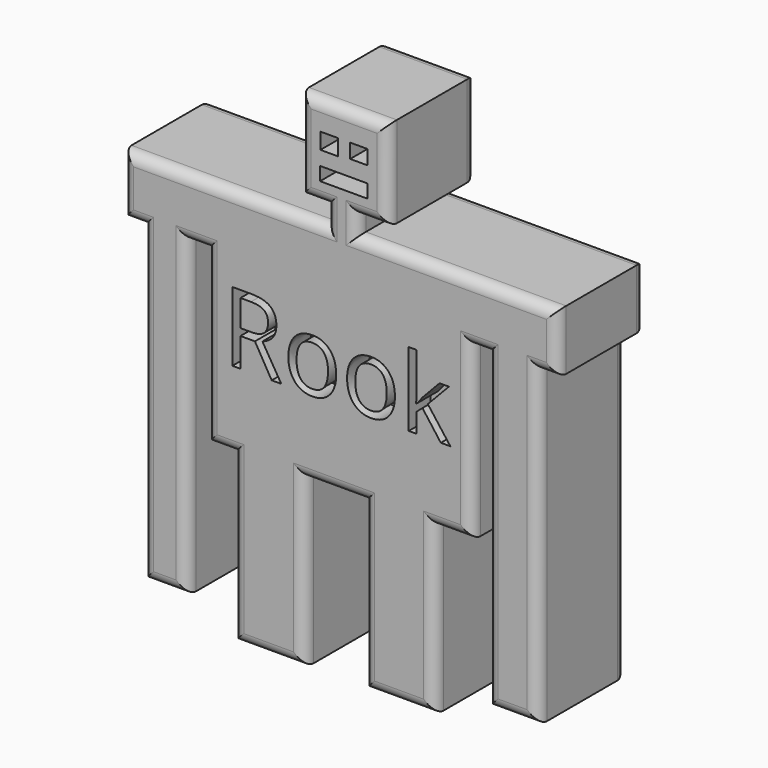
from build123d import *

# Parameters (mm, degrees)
F0_W         = 7.1803850587
F0_H         = 4.1030719876
F0_W_2       = 10.2576911449
F0_H_2       = 72.1457730979
F0_W_3       = 11.7963477969
F0_W_4       = 16.5832703933
F0_H_3       = 38.4663501754
F0_W_5       = 16.4123084396
F0_H_4       = 38.2953854278
F1_DEPTH     = 25.4
F2_R         = 2.54
F3_TEXT_SIZE = 22.484323967
F4_DEPTH     = 6.35
F5_W         = 4.116662778
F5_H         = 3.7231482565
F5_W_2       = 4.0594090242
F5_H_2       = 3.3319927752
F5_W_3       = 10.9823788516
F5_H_3       = 3.1074360013
F6_DEPTH     = 6.35


# Not quite as in the source:
# - a length typed as a fraction of an inch, garbled in the dataset ("3 / 203.2 mm" for 3/8 in), is restored
# - Text() gives the source's letters only with a copy of the font that has no kerning and outlines rounded to 1/6400 em; it was checked with that copy


with BuildPart() as f1:
    # F0 (on Front) → F1 (new body)
    with BuildSketch(Plane.XZ):
        Polygon((11.5399044007, 63.8541355729), (-8.8045196608, 63.8541355729), (-8.8045196608, 42.8258627653), (-2.820865484, 42.8258627653), (4.3595195748, 42.8258627653), (11.5399044007, 42.8258627653), align=None)
        with Locations((0.7693270454, 40.7743267715)):
            Rectangle(F0_W, F0_H)
        Polygon((4.3595195748, 38.7227907777), (-2.820865484, 38.7227907777), (-30.5166337639, 38.7227907777), (-30.5166337639, 24.8749051243), (-30.5166337639, -14.6172111854), (-24.3620201945, -14.6172111854), (-7.7787498012, -14.6172111854), (5.8981720358, -14.6172111854), (22.3104804754, -14.6172111854), (30.858559534, -14.6172111854), (30.858559534, 24.8749051243), (30.858559534, 38.7227907777), align=None)
        Polygon((-30.5166337639, 24.8749051243), (-30.5166337639, 38.7227907777), (-49.8352870345, 38.7227907777), (-49.8352870345, 24.8749051243), (-45.2193245292, 24.8749051243), (-34.9616333842, 24.8749051243), align=None)
        Polygon((50.6900958717, 38.7227907777), (30.858559534, 38.7227907777), (30.858559534, 24.8749051243), (34.4487503171, 24.8749051243), (46.245098114, 24.8749051243), (50.6900958717, 24.8749051243), align=None)
        with Locations((-40.0904789567, -11.1979814246)):
            Rectangle(F0_W_2, F0_H_2)
        with Locations((40.3469242156, -11.1979814246)):
            Rectangle(F0_W_3, F0_H_2)
        with Locations((-16.0703849979, -33.8503862731)):
            Rectangle(F0_W_4, F0_H_3)
        with Locations((14.1043262556, -33.7649038993)):
            Rectangle(F0_W_5, F0_H_4)
    extrude(amount=-F1_DEPTH)

    # F2
    f2_edges = [f1.edges().sort_by_distance(p)[0] for p in [
        (1.367692, 0, 63.854136),
        (-8.80452, 0, 53.339999),
        (-5.812693, 0, 42.825863),
        (-2.820865, 0, 40.774327),
        (-26.328076, 0, 38.722791),
        (-49.835287, 0, 31.798848),
        (-47.527306, 0, 24.874905),
        (-45.219325, 0, -11.197981),
        (-40.090479, 0, -47.270868),
        (-34.961633, 0, -11.197981),
        (-32.739134, 0, 24.874905),
        (-30.516634, 0, 5.128847),
        (-27.439327, 0, -14.617211),
        (-24.36202, 0, -33.850386),
        (-16.070385, 0, -53.083561),
        (-7.77875, 0, -33.850386),
        (-0.940289, 0, -14.617211),
        (5.898172, 0, -33.764904),
        (14.104326, 0, -52.912597),
        (22.31048, 0, -33.764904),
        (26.58452, 0, -14.617211),
        (30.85856, 0, 5.128847),
        (32.653655, 0, 24.874905),
        (34.44875, 0, -11.197981),
        (40.346924, 0, -47.270868),
        (46.245098, 0, -11.197981),
        (48.467597, 0, 24.874905),
        (50.690096, 0, 31.798848),
        (27.524808, 0, 38.722791),
        (4.35952, 0, 40.774327),
        (7.949712, 0, 42.825863),
        (11.539904, 0, 53.339999),
        (11.539904, 25.4, 53.339999),
        (-8.80452, 25.4, 53.339999),
        (1.367692, 25.4, 63.854136),
        (27.524808, 25.4, 38.722791),
        (50.690096, 25.4, 31.798848),
        (48.467597, 25.4, 24.874905),
        (46.245098, 25.4, -11.197981),
        (40.346924, 25.4, -47.270868),
        (34.44875, 25.4, -11.197981),
        (32.653655, 25.4, 24.874905),
        (30.85856, 25.4, 5.128847),
        (22.31048, 25.4, -33.764904),
        (14.104326, 25.4, -52.912597),
        (5.898172, 25.4, -33.764904),
        (-16.070385, 25.4, -53.083561),
        (-24.36202, 25.4, -33.850386),
        (-27.439327, 25.4, -14.617211),
        (-30.516634, 25.4, 5.128847),
        (-32.739134, 25.4, 24.874905),
        (-40.090479, 25.4, -47.270868),
        (-45.219325, 25.4, -11.197981),
        (-2.820865, 25.4, 40.774327),
        (-26.328076, 25.4, 38.722791),
        (-34.961633, 25.4, -11.197981),
        (-7.77875, 25.4, -33.850386),
        (26.58452, 25.4, -14.617211),
        (-49.835287, 25.4, 31.798848),
        (4.35952, 25.4, 40.774327),
        (-47.527306, 25.4, 24.874905),
        (7.949712, 25.4, 42.825863),
        (-5.812693, 25.4, 42.825863),
        (-0.940289, 25.4, -14.617211),
    ]]
    fillet(f2_edges, radius=F2_R)

    # F3 (on Front) → F4 (cut)
    with BuildSketch(Plane.XZ):
        with Locations((-26.6869510524, 3.1131892465)):
            Text('Rook', F3_TEXT_SIZE, font='Open Sans', text_align=(TextAlign.LEFT, TextAlign.BOTTOM))
    extrude(amount=-F4_DEPTH, mode=Mode.SUBTRACT)

    # F5 (on Front) → F6 (cut)
    with BuildSketch(Plane.XZ):
        with Locations((-2.058331389, 55.5552970618)):
            Rectangle(F5_W, F5_H)
        with Locations((4.7946962295, 55.7508748025)):
            Rectangle(F5_W_2, F5_H_2)
        with Locations((1.2927257922, 48.847541213)):
            Rectangle(F5_W_3, F5_H_3)
    extrude(amount=-F6_DEPTH, mode=Mode.SUBTRACT)


solid = f1.part
